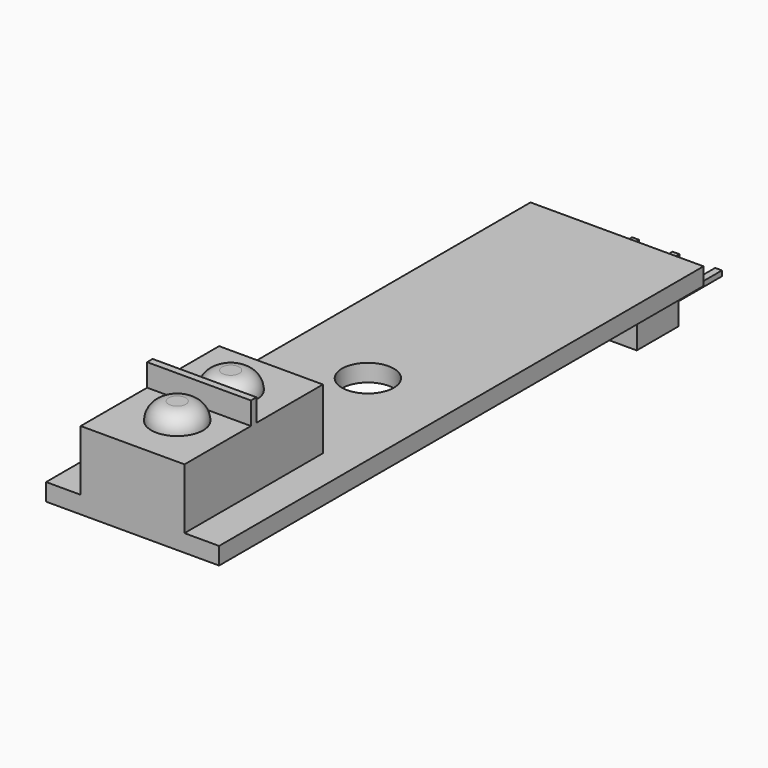
from build123d import *

# Parameters (mm, degrees)
F0_W      = 10
F0_H      = 35
F1_DEPTH  = 1
F2_W      = 6
F2_H      = 10
F3_DEPTH  = 3.5
F4_R      = 1.5
F5_DEPTH  = 1
F6_W      = 8.476907853
F6_H      = 3.0214712024
F7_DEPTH  = 2
F8_W      = 0.392
F8_H      = 7
F9_DEPTH  = 0.3
F10_R     = 1.5
F11_DEPTH = 3.301
F12_R     = 0.99999
F13_W     = 6
F13_H     = 0.4
F14_DEPTH = 1.3


# Not quite as in the source:
# - a fillet or chamfer is up to 0.001 mm smaller than in the source, because OpenCascade refuses the exact size


with BuildPart() as f1:
    # F0 (on Top) → F1 (new body)
    with BuildSketch(Plane.XY):
        with Locations((-11.4876428805, 10.5133079179)):
            Rectangle(F0_W, F0_H)
    extrude(amount=F1_DEPTH)

    # F2 (on face) → F3 (join)
    with BuildSketch(Plane.XY.offset(1)):
        with Locations((-11.4876428805, -1.9866920821)):
            Rectangle(F2_W, F2_H)
    extrude(amount=F3_DEPTH)

    # F4 (on face) → F5 (join)
    with BuildSketch(Plane.XY.offset(4.5)):
        with Locations((-11.4072084332, 0)):
            Circle(F4_R)
        with Locations((-11.4072084332, -3.8623050655)):
            Circle(F4_R)
    extrude(amount=F5_DEPTH)

    # F6 (on face) → F7 (join)
    with BuildSketch(Plane(origin=(0, 0, 0), x_dir=(1, 0, 0), z_dir=(0, 0, -1))):
        with Locations((-11.5416448098, -25.7204081863)):
            Rectangle(F6_W, F6_H)
    extrude(amount=F7_DEPTH)

    # F8 (on face) → F9 (join)
    with BuildSketch(Plane(origin=(0, 0, -2), x_dir=(1, 0, 0), z_dir=(0, 0, -1))):
        with Locations((-14.1843358078, -29.2204081863)):
            Rectangle(F8_W, F8_H)
        with Locations((-11.8782826397, -29.261767303)):
            Rectangle(F8_W, F8_H)
        with Locations((-9.3856059038, -29.2204081863)):
            Rectangle(F8_W, F8_H)
    extrude(amount=F9_DEPTH)

    # F10 (on face) → F11 (cut, through all)
    with BuildSketch(Plane.XY.offset(1)):
        with Locations((-11.4876428805, 10.0133079179)):
            Circle(F10_R)
    extrude(amount=-F11_DEPTH, mode=Mode.SUBTRACT)

    # F12 (radius 1 in the source; OpenCascade refuses exactly that, so slightly less here)
    f12_edges = [f1.edges().sort_by_distance(p)[0] for p in [
        (-12.907208, -3.862305, 5.5),
        (-12.907208, 0, 5.5),
    ]]
    fillet(f12_edges, radius=F12_R)

    # F13 (on face) → F14 (join)
    with BuildSketch(Plane.XY.offset(4.5)):
        with Locations((-11.4876428805, -1.9866920821)):
            Rectangle(F13_W, F13_H)
    extrude(amount=F14_DEPTH)


solid = f1.part
